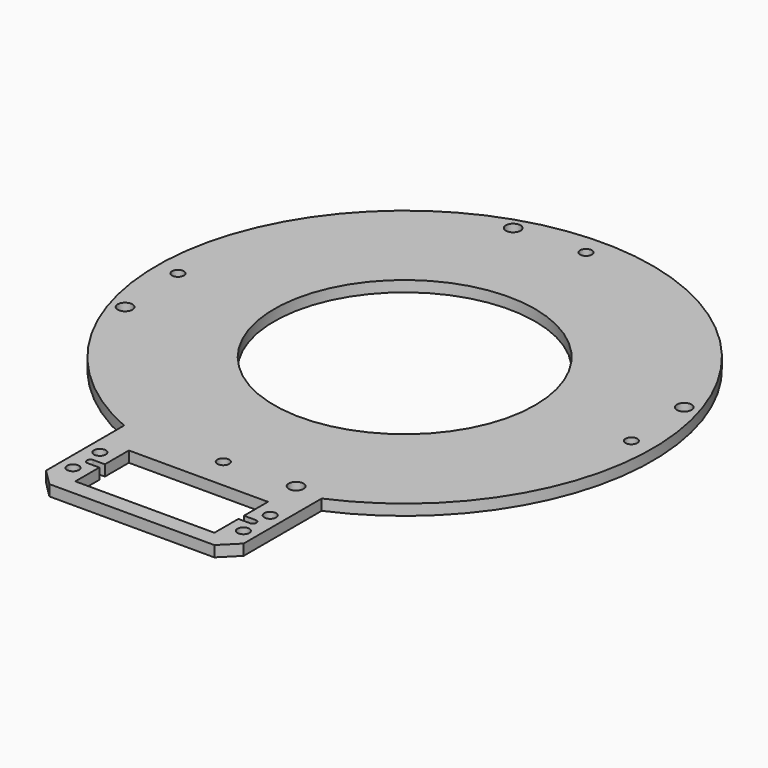
from build123d import *

# Parameters (mm, degrees)
F0_R     = 1.7272
F0_R_2   = 2.15265
F0_R_3   = 38.1
F1_DEPTH = 3.175
F2_SIZE  = 4.7625


# Not quite as in the source:
# - a feature names something its author has since deleted; it is built from what else it names


with BuildPart() as f1:
    # F0 (on Top) → F1 (new body)
    with BuildSketch(Plane.XY):
        with BuildLine():
            Line((28.86075, -99.6367724936), (28.86075, -66.3880200747))
            ThreePointArc((28.86075, -66.3880200747), (0, 72.39), (-28.86075, -66.3880200747))
            Line((-28.86075, -66.3880200747), (-28.86075, -99.6367724936))
            Line((-28.86075, -99.6367724936), (28.86075, -99.6367724936))
        make_face()
        with Locations((-24.892, -89.9847724936)):
            Circle(F0_R, mode=Mode.SUBTRACT)
        with Locations((-24.892, -80.2057724936)):
            Circle(F0_R, mode=Mode.SUBTRACT)
        with Locations((-65.2747423649, -20.5103744665)):
            Circle(F0_R_2, mode=Mode.SUBTRACT)
        with BuildLine():
            Line((-20.32, -94.8742724936), (-20.32, -86.1112724936))
            Line((-20.32, -86.1112724936), (-23.749, -86.1112724936))
            ThreePointArc((-23.749, -86.1112724936), (-24.765, -85.0952724936), (-23.749, -84.0792724936))
            Line((-23.749, -84.0792724936), (-20.32, -84.0792724936))
            Line((-20.32, -84.0792724936), (-20.32, -75.3162724936))
            Line((-20.32, -75.3162724936), (20.32, -75.3162724936))
            Line((20.32, -75.3162724936), (20.32, -84.0792724936))
            Line((20.32, -84.0792724936), (23.749, -84.0792724936))
            ThreePointArc((23.749, -84.0792724936), (24.765, -85.0952724936), (23.749, -86.1112724936))
            Line((23.749, -86.1112724936), (20.32, -86.1112724936))
            Line((20.32, -86.1112724936), (20.32, -94.8742724936))
            Line((20.32, -94.8742724936), (-20.32, -94.8742724936))
        make_face(mode=Mode.SUBTRACT)
        with Locations((24.892, -89.9847724936)):
            Circle(F0_R, mode=Mode.SUBTRACT)
        with Locations((24.892, -80.2057724936)):
            Circle(F0_R, mode=Mode.SUBTRACT)
        with Locations((0, -66.2293888929)):
            Circle(F0_R, mode=Mode.SUBTRACT)
        with Locations((20.5103744665, -65.2747423649)):
            Circle(F0_R_2, mode=Mode.SUBTRACT)
        with Locations((-66.2293888929, 0)):
            Circle(F0_R, mode=Mode.SUBTRACT)
        with Locations((-20.5103744665, 65.2747423649)):
            Circle(F0_R_2, mode=Mode.SUBTRACT)
        Circle(F0_R_3, mode=Mode.SUBTRACT)
        with Locations((66.2293888929, 0)):
            Circle(F0_R, mode=Mode.SUBTRACT)
        with Locations((65.2747423649, 20.5103744665)):
            Circle(F0_R_2, mode=Mode.SUBTRACT)
        with Locations((0, 66.2293888929)):
            Circle(F0_R, mode=Mode.SUBTRACT)
    extrude(amount=F1_DEPTH)

    # F2
    f2_edges = [f1.edges().sort_by_distance(p)[0] for p in [
        (-28.86075, -99.636772, 1.5875),
        (28.86075, -99.636772, 1.5875),
    ]]
    chamfer(f2_edges, length=F2_SIZE)


solid = f1.part
